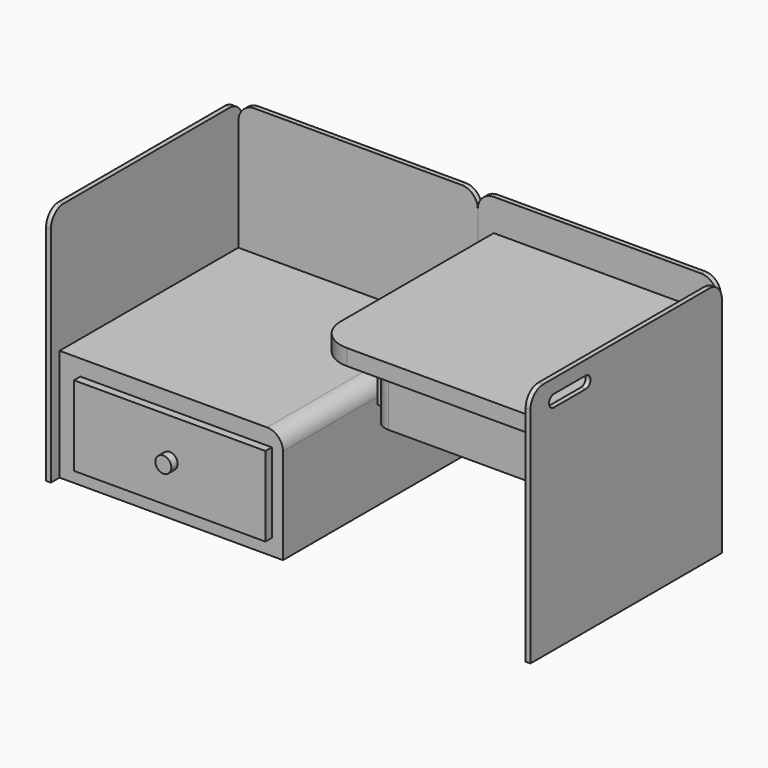
from build123d import *

# Parameters (mm, degrees)
F0_W      = 38.1
F0_H      = 38.1
F2_DEPTH  = 0.762
F1_W      = 38.1
F1_H      = 38.1
F3_DEPTH  = 0.762
F4_W      = 35.56
F4_H      = 35.56
F5_DEPTH  = 17.78
F8_W      = 30.48
F8_H      = 30.48
F9_DEPTH  = 10.16
F7_W      = 35.56
F7_H      = 35.56
F10_DEPTH = 2.54
F11_W     = 30.48
F11_H     = 12.7
F12_DEPTH = 1.27
F13_R     = 1.27
F14_DEPTH = 1.27
F16_R     = 1.27
F17_DEPTH = 2.54
F15_W     = 25.4
F15_H     = 7.62
F18_DEPTH = 1.27
F19_R     = 2.54
F19_2_R   = 2.54
F19_3_R   = 2.54
F19_4_R   = 2.54
F20_R     = 5.08
F23_DEPTH = 12.7
F24_DEPTH = 0.762
F26_W     = 38.1
F26_H     = 38.1
F27_DEPTH = 0.762
F29_DEPTH = 12.7
F30_R     = 2.54
F30_2_R   = 2.54


# Not quite as in the source:
# - two fillets or chamfers of one size are made in one step
# - a feature names something its author has since deleted; it is built from what else it names


with BuildPart() as f2:
    # F0 (on Right) → F2 (new body)
    with BuildSketch(Plane.YZ):
        with Locations((-19.05, 19.05)):
            Rectangle(F0_W, F0_H)
    extrude(amount=-F2_DEPTH)

    # F19
    f19_edges = [f2.edges().sort_by_distance(p)[0] for p in [
        (-0.381, -38.1, 38.1),
        (-0.381, 0, 38.1),
    ]]
    fillet(f19_edges, radius=F19_R)

    # F22 (on face) → F23 (cut)
    with BuildSketch(Plane.YZ):
        with BuildLine():
            ThreePointArc((35.283215344, 34.4806989491), (34.330715344, 35.4331989491), (33.378215344, 34.4806989491))
            Line((33.378215344, 34.4806989491), (33.378215344, 28.1306989491))
            ThreePointArc((33.378215344, 28.1306989491), (34.330715344, 27.1781989491), (35.283215344, 28.1306989491))
            Line((35.283215344, 28.1306989491), (35.283215344, 34.4806989491))
        make_face()
    extrude(amount=-F23_DEPTH, mode=Mode.SUBTRACT)


with BuildPart() as f3:
    # F1 (on Front) → F3 (new body)
    with BuildSketch(Plane.XZ):
        with Locations((19.05, 19.05)):
            Rectangle(F1_W, F1_H)
    extrude(amount=F3_DEPTH)

    # F19#2
    f19_2_edges = [f3.edges().sort_by_distance(p)[0] for p in [
        (0, -0.381, 38.1),
        (38.1, -0.381, 38.1),
    ]]
    fillet(f19_2_edges, radius=F19_2_R)


with BuildPart() as f5:
    # F4 (on Top) → F5 (new body)
    with BuildSketch(Plane.XY):
        with Locations((17.78, -18.5785688174)):
            Rectangle(F4_W, F4_H)
    extrude(amount=F5_DEPTH)

    # F19#3
    f19_3_edges = [f5.edges().sort_by_distance(p)[0] for p in [
        (35.56, -18.578569, 17.78),
    ]]
    fillet(f19_3_edges, radius=F19_3_R)


with BuildPart() as f9:
    # F8 (on offset) → F9 (new body)
    with BuildSketch(Plane.XY.offset(30.48)):
        with Locations((60.96, -16.002)):
            Rectangle(F8_W, F8_H)
    extrude(amount=-F9_DEPTH)

    # F19#4
    f19_4_edges = [f9.edges().sort_by_distance(p)[0] for p in [
        (45.72, -31.242, 25.4),
    ]]
    fillet(f19_4_edges, radius=F19_4_R)


with BuildPart() as f10:
    # F7 (on offset) → F10 (new body)
    with BuildSketch(Plane.XY.offset(30.48)):
        with Locations((58.42, -18.542)):
            Rectangle(F7_W, F7_H)
    extrude(amount=F10_DEPTH)

    # F20
    f20_edges = [f10.edges().sort_by_distance(p)[0] for p in [
        (40.64, -36.322, 31.75),
    ]]
    fillet(f20_edges, radius=F20_R)


with BuildPart() as f12:
    # F11 (on face) → F12 (new body)
    with BuildSketch(Plane.XZ.offset(36.3585688174)):
        with Locations((18.542, 8.89)):
            Rectangle(F11_W, F11_H)
    extrude(amount=F12_DEPTH)


with BuildPart() as f14:
    # F13 (on face) → F14 (new body)
    with BuildSketch(Plane.XZ.offset(37.6285688174)):
        with Locations((18.542, 8.89)):
            Circle(F13_R)
    extrude(amount=F14_DEPTH)


with BuildPart() as f17:
    # F16 (on face) → F17 (new body)
    with BuildSketch(Plane(origin=(45.72, 0, 0), x_dir=(0, -1, 0), z_dir=(-1, 0, 0))):
        with Locations((16.002, 25.4)):
            Circle(F16_R)
    extrude(amount=F17_DEPTH)


with BuildPart() as f18:
    # F15 (on face) → F18 (new body)
    with BuildSketch(Plane(origin=(45.72, 0, 0), x_dir=(0, -1, 0), z_dir=(-1, 0, 0))):
        with Locations((16.002, 25.4)):
            Rectangle(F15_W, F15_H)
    extrude(amount=F18_DEPTH)


with BuildPart() as f24:
    # F1 (on Front) → F24 (new body)
    with BuildSketch(Plane.XZ):
        with Locations((57.15, 19.05)):
            Rectangle(F1_W, F1_H)
    extrude(amount=F24_DEPTH)

    # F30
    f30_edges = [f24.edges().sort_by_distance(p)[0] for p in [
        (76.2, -0.381, 38.1),
        (38.1, -0.381, 38.1),
    ]]
    fillet(f30_edges, radius=F30_R)


with BuildPart() as f27:
    # F26 (on offset) → F27 (new body)
    with BuildSketch(Plane.YZ.offset(76.2)):
        with Locations((-19.812, 19.05)):
            Rectangle(F26_W, F26_H)
    extrude(amount=F27_DEPTH)

    # F28 (on face) → F29 (cut)
    with BuildSketch(Plane.YZ.offset(76.962)):
        with BuildLine():
            Line((-27.8631728142, 35.8923991907), (-34.2131728142, 35.8923991907))
            ThreePointArc((-34.2131728142, 35.8923991907), (-35.1656728142, 34.9398991907), (-34.2131728142, 33.9873991907))
            Line((-34.2131728142, 33.9873991907), (-27.8631728142, 33.9873991907))
            ThreePointArc((-27.8631728142, 33.9873991907), (-26.9106728142, 34.9398991907), (-27.8631728142, 35.8923991907))
        make_face()
    extrude(amount=-F29_DEPTH, mode=Mode.SUBTRACT)

    # F30#2
    f30_2_edges = [f27.edges().sort_by_distance(p)[0] for p in [
        (76.581, -0.762, 38.1),
        (76.581, -38.862, 38.1),
    ]]
    fillet(f30_2_edges, radius=F30_2_R)


solid = Compound([f2.part, f3.part, f5.part, f9.part, f10.part, f12.part, f14.part, f17.part, f18.part, f24.part, f27.part])
